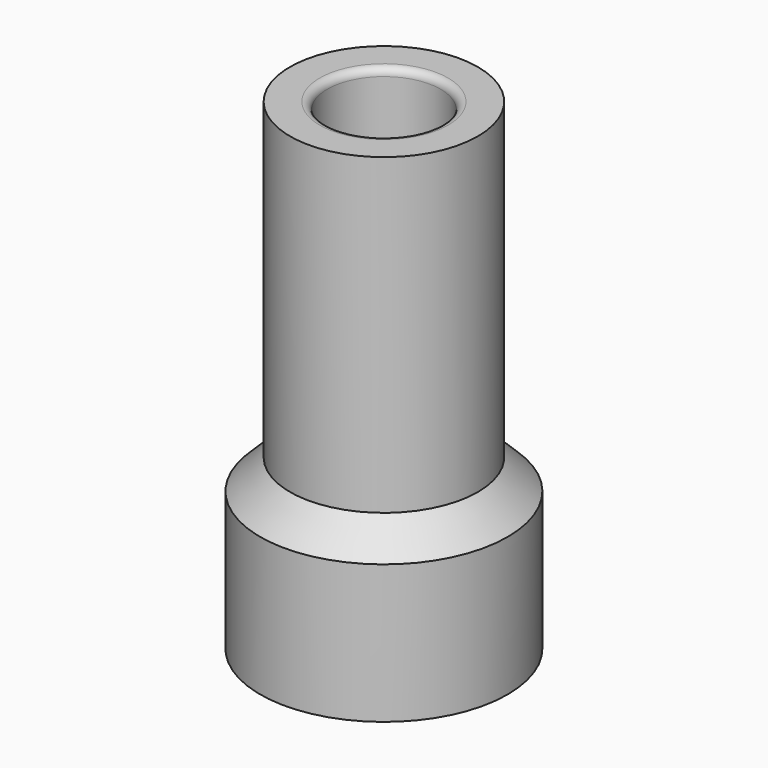
from build123d import *

# Parameters (mm, degrees)
F0_R          = 6.3
F0_R_2        = 3.8
F1_DEPTH      = 25
F2_R          = 8.3
F2_R_2        = 6.3
F3_DEPTH      = 7.3
F3_DEPTH_BACK = 2
F4_SIZE       = 1.99999
F5_R          = 0.5


# Not quite as in the source:
# - a fillet or chamfer is up to 0.001 mm smaller than in the source, because OpenCascade refuses the exact size


with BuildPart() as f1:
    # F0 (on Top) → F1 (new body)
    with BuildSketch(Plane.XY):
        Circle(F0_R)
        Circle(F0_R_2, mode=Mode.SUBTRACT)
    extrude(amount=F1_DEPTH)

    # F2 (on face) → F3 (join, two sides)
    with BuildSketch(Plane(origin=(0, 0, 0), x_dir=(1, 0, 0), z_dir=(0, 0, -1))) as f3_sk:
        Circle(F2_R)
        Circle(F2_R_2, mode=Mode.SUBTRACT)
    extrude(amount=F3_DEPTH)
    extrude(f3_sk.sketch, amount=-F3_DEPTH_BACK)

    # F4 (size 2 in the source; OpenCascade refuses exactly that, so slightly less here)
    f4_edges = [f1.edges().sort_by_distance(p)[0] for p in [
        (-6.3, 0, 2),
    ]]
    chamfer(f4_edges, length=F4_SIZE)

    # F5
    f5_edges = [f1.edges().sort_by_distance(p)[0] for p in [
        (-3.8, 0, 25),
        (-6.3, 0, -7.3),
    ]]
    fillet(f5_edges, radius=F5_R)


solid = f1.part
